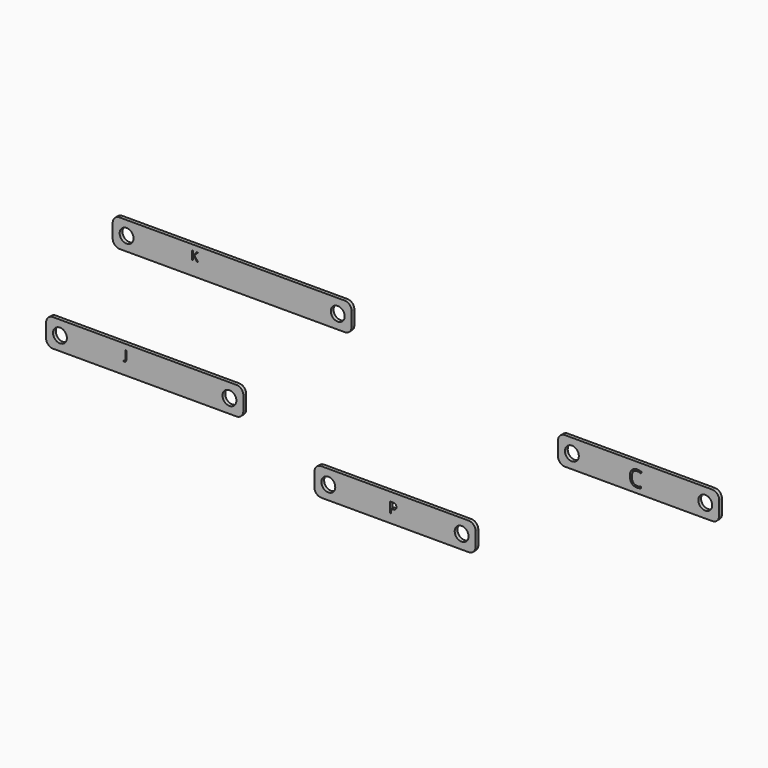
from build123d import *

# Parameters (mm, degrees)
F1_R     = 6.35
F2_DEPTH = 3.175
F3_R     = 6.35
F4_DEPTH = 3.175
F5_R     = 6.35
F6_DEPTH = 3.175
F7_R     = 6.35
F8_DEPTH = 3.175


# Not quite as in the source:
# - a length typed as a fraction of an inch, garbled in the dataset ("3 / 203.2 mm" for 3/8 in), is restored


with BuildPart() as f2:
    # F1 (on Front) → F2 (new body)
    with BuildSketch(Plane.XZ):
        with BuildLine():
            Line((95.5763677621, 23.3495529922), (-110.1636322379, 23.3495529922))
            ThreePointArc((-110.1636322379, 23.3495529922), (-114.6537602984, 21.4896810527), (-116.5136322379, 16.9995529922))
            Line((-116.5136322379, 16.9995529922), (-116.5136322379, 4.2995529922))
            ThreePointArc((-116.5136322379, 4.2995529922), (-114.6537602984, -0.1905750684), (-110.1636322379, -2.0504470078))
            Line((-110.1636322379, -2.0504470078), (95.5763677621, -2.0504470078))
            ThreePointArc((95.5763677621, -2.0504470078), (100.0664958226, -0.1905750684), (101.9263677621, 4.2995529922))
            Line((101.9263677621, 4.2995529922), (101.9263677621, 16.9995529922))
            ThreePointArc((101.9263677621, 16.9995529922), (100.0664958226, 21.4896810527), (95.5763677621, 23.3495529922))
        make_face()
        with Locations((-103.8136322379, 10.6495529922)):
            Circle(F1_R, mode=Mode.SUBTRACT)
        Polygon((-41.6826481417, 14.9866065492), (-38.4835676154, 10.6495529922), (-39.5325840524, 10.6495529922), (-42.3271638406, 14.3689456712), (-43.1311300379, 13.655614494), (-43.1311300379, 10.6495529922), (-44.0223744027, 10.6495529922), (-44.0223744027, 18.3182827531), (-43.1311300379, 18.3182827531), (-43.1311300379, 14.5149687592), (-39.653430746, 18.3182827531), (-38.5993790301, 18.3182827531), align=None, mode=Mode.SUBTRACT)
        with Locations((89.2263677621, 10.6495529922)):
            Circle(F1_R, mode=Mode.SUBTRACT)
    extrude(amount=F2_DEPTH)


with BuildPart() as f4:
    # F3 (on Front) → F4 (new body)
    with BuildSketch(Plane.XZ):
        with BuildLine():
            Line((-3.4336355138, -76.6887728453), (-171.0736355138, -76.6887728453))
            ThreePointArc((-171.0736355138, -76.6887728453), (-175.5637635743, -78.5486447847), (-177.4236355138, -83.0387728453))
            Line((-177.4236355138, -83.0387728453), (-177.4236355138, -95.7387728453))
            ThreePointArc((-177.4236355138, -95.7387728453), (-175.5637635743, -100.2289009058), (-171.0736355138, -102.0887728453))
            Line((-171.0736355138, -102.0887728453), (-3.4336355138, -102.0887728453))
            ThreePointArc((-3.4336355138, -102.0887728453), (1.0564925468, -100.2289009058), (2.9163644862, -95.7387728453))
            Line((2.9163644862, -95.7387728453), (2.9163644862, -83.0387728453))
            ThreePointArc((2.9163644862, -83.0387728453), (1.0564925468, -78.5486447847), (-3.4336355138, -76.6887728453))
        make_face()
        with Locations((-9.7836355138, -89.3887728453)):
            Circle(F3_R, mode=Mode.SUBTRACT)
        with Locations((-164.7236355138, -89.3887728453)):
            Circle(F3_R, mode=Mode.SUBTRACT)
        with BuildLine():
            add(Edge.make_bspline(
                [(-104.6017276977, -90.8599134965), (-105.1052555874, -91.4079196832), (-106.0502095939, -91.4079196832)],
                knots=[0, 0, 0, 1, 1, 1], degree=2))
            add(Edge.make_bspline(
                [(-106.0502095939, -91.4079196832), (-106.5419884995, -91.4079196832), (-106.8256425441, -91.266931874)],
                knots=[0, 0, 0, 1, 1, 1], degree=2))
            Line((-106.8256425441, -91.266931874), (-106.8256425441, -90.5066047605))
            add(Edge.make_bspline(
                [(-106.8256425441, -90.5066047605), (-106.4530319057, -90.6106671911), (-106.0502095939, -90.6106671911)],
                knots=[0, 0, 0, 1, 1, 1], degree=2))
            add(Edge.make_bspline(
                [(-106.0502095939, -90.6106671911), (-105.5298974411, -90.6106671911), (-105.2596708069, -90.29596226)],
                knots=[0, 0, 0, 1, 1, 1], degree=2))
            add(Edge.make_bspline(
                [(-105.2596708069, -90.29596226), (-104.9894441728, -89.9812573289), (-104.9894441728, -89.3887728453)],
                knots=[0, 0, 0, 1, 1, 1], degree=2))
            Line((-104.9894441728, -89.3887728453), (-104.9894441728, -81.7200430843))
            Line((-104.9894441728, -81.7200430843), (-104.0981998079, -81.7200430843))
            Line((-104.0981998079, -81.7200430843), (-104.0981998079, -89.3149220881))
            add(Edge.make_bspline(
                [(-104.0981998079, -89.3149220881), (-104.0981998079, -90.3119073098), (-104.6017276977, -90.8599134965)],
                knots=[0, 0, 0, 1, 1, 1], degree=2))
        make_face(mode=Mode.SUBTRACT)
    extrude(amount=F4_DEPTH)


with BuildPart() as f6:
    # F5 (on Front) → F6 (new body)
    with BuildSketch(Plane.XZ):
        with BuildLine():
            Line((208.8844542503, -116.8920610428), (74.2644542503, -116.8920610428))
            ThreePointArc((74.2644542503, -116.8920610428), (69.7743261898, -118.7519329823), (67.9144542503, -123.2420610428))
            Line((67.9144542503, -123.2420610428), (67.9144542503, -135.9420610428))
            ThreePointArc((67.9144542503, -135.9420610428), (69.7743261898, -140.4321891033), (74.2644542503, -142.2920610428))
            Line((74.2644542503, -142.2920610428), (208.8844542503, -142.2920610428))
            ThreePointArc((208.8844542503, -142.2920610428), (213.3745823109, -140.4321891033), (215.2344542503, -135.9420610428))
            Line((215.2344542503, -135.9420610428), (215.2344542503, -123.2420610428))
            ThreePointArc((215.2344542503, -123.2420610428), (213.3745823109, -118.7519329823), (208.8844542503, -116.8920610428))
        make_face()
        with Locations((202.5344542503, -129.5920610428)):
            Circle(F5_R, mode=Mode.SUBTRACT)
        with Locations((80.6144542503, -129.5920610428)):
            Circle(F5_R, mode=Mode.SUBTRACT)
        with BuildLine():
            add(Edge.make_bspline(
                [(139.3608329236, -124.7941682377), (142.9005294922, -124.7941682377), (142.9005294922, -127.5461169134)],
                knots=[0, 0, 0, 1, 1, 1], degree=2))
            add(Edge.make_bspline(
                [(142.9005294922, -127.5461169134), (142.9005294922, -128.9810172748), (141.9215304704, -129.7532583194)],
                knots=[0, 0, 0, 1, 1, 1], degree=2))
            add(Edge.make_bspline(
                [(141.9215304704, -129.7532583194), (140.9425314487, -130.525499364), (139.1209936701, -130.525499364)],
                knots=[0, 0, 0, 1, 1, 1], degree=2))
            Line((139.1209936701, -130.525499364), (138.0086357531, -130.525499364))
            Line((138.0086357531, -130.525499364), (138.0086357531, -134.2409402132))
            Line((138.0086357531, -134.2409402132), (136.9107508945, -134.2409402132))
            Line((136.9107508945, -134.2409402132), (136.9107508945, -124.7941682377))
            Line((136.9107508945, -124.7941682377), (139.3608329236, -124.7941682377))
        make_face(mode=Mode.SUBTRACT)
    extrude(amount=F6_DEPTH)


with BuildPart() as f8:
    # F7 (on Front) → F8 (new body)
    with BuildSketch(Plane.XZ):
        with BuildLine():
            Line((431.5898662186, -19.4524478495), (296.9698662186, -19.4524478495))
            ThreePointArc((296.9698662186, -19.4524478495), (292.479738158, -21.312319789), (290.6198662186, -25.8024478495))
            Line((290.6198662186, -25.8024478495), (290.6198662186, -38.5024478495))
            ThreePointArc((290.6198662186, -38.5024478495), (292.479738158, -42.99257591), (296.9698662186, -44.8524478495))
            Line((296.9698662186, -44.8524478495), (431.5898662186, -44.8524478495))
            ThreePointArc((431.5898662186, -44.8524478495), (436.0799942791, -42.99257591), (437.9398662186, -38.5024478495))
            Line((437.9398662186, -38.5024478495), (437.9398662186, -25.8024478495))
            ThreePointArc((437.9398662186, -25.8024478495), (436.0799942791, -21.312319789), (431.5898662186, -19.4524478495))
        make_face()
        with BuildLine():
            add(Edge.make_bspline(
                [(366.4639369183, -27.8038420737), (364.8282573372, -27.0380036572), (363.1925777562, -27.0380036572)],
                knots=[0, 0, 0, 1, 1, 1], degree=2))
            add(Edge.make_bspline(
                [(363.1925777562, -27.0380036572), (360.8194241444, -27.0380036572), (359.4453272324, -28.6185302658)],
                knots=[0, 0, 0, 1, 1, 1], degree=2))
            add(Edge.make_bspline(
                [(359.4453272324, -28.6185302658), (358.0712303204, -30.1990568745), (358.0712303204, -32.9472506985)],
                knots=[0, 0, 0, 1, 1, 1], degree=2))
            add(Edge.make_bspline(
                [(358.0712303204, -32.9472506985), (358.0712303204, -35.7710828846), (359.3964774569, -37.3137903122)],
                knots=[0, 0, 0, 1, 1, 1], degree=2))
            add(Edge.make_bspline(
                [(359.3964774569, -37.3137903122), (360.7217245933, -38.8564977398), (363.1736681657, -38.8564977398)],
                knots=[0, 0, 0, 1, 1, 1], degree=2))
            add(Edge.make_bspline(
                [(363.1736681657, -38.8564977398), (364.6801322114, -38.8564977398), (366.6120620441, -38.3144228112)],
                knots=[0, 0, 0, 1, 1, 1], degree=2))
            Line((366.6120620441, -38.3144228112), (366.6120620441, -39.7799160775))
            add(Edge.make_bspline(
                [(366.6120620441, -39.7799160775), (365.1150527937, -40.344052195), (362.9183886935, -40.344052195)],
                knots=[0, 0, 0, 1, 1, 1], degree=2))
            add(Edge.make_bspline(
                [(362.9183886935, -40.344052195), (359.7384258857, -40.344052195), (358.0097741512, -38.4121223623)],
                knots=[0, 0, 0, 1, 1, 1], degree=2))
            add(Edge.make_bspline(
                [(358.0097741512, -38.4121223623), (356.2811224167, -36.4801925296), (356.2811224167, -32.9251895095)],
                knots=[0, 0, 0, 1, 1, 1], degree=2))
            add(Edge.make_bspline(
                [(356.2811224167, -32.9251895095), (356.2811224167, -30.7001610236), (357.1131444001, -29.0266622615)],
                knots=[0, 0, 0, 1, 1, 1], degree=2))
            add(Edge.make_bspline(
                [(357.1131444001, -29.0266622615), (357.9451663835, -27.3531634994), (359.5162381969, -26.447078953)],
                knots=[0, 0, 0, 1, 1, 1], degree=2))
            add(Edge.make_bspline(
                [(359.5162381969, -26.447078953), (361.0873100103, -25.5409944067), (363.2146389452, -25.5409944067)],
                knots=[0, 0, 0, 1, 1, 1], degree=2))
            add(Edge.make_bspline(
                [(363.2146389452, -25.5409944067), (365.4774866122, -25.5409944067), (367.1730465632, -26.3667131933)],
                knots=[0, 0, 0, 1, 1, 1], degree=2))
            Line((367.1730465632, -26.3667131933), (366.4639369183, -27.8038420737))
        make_face(mode=Mode.SUBTRACT)
        with Locations((425.2398662186, -32.1524478495)):
            Circle(F7_R, mode=Mode.SUBTRACT)
        with Locations((303.3198662186, -32.1524478495)):
            Circle(F7_R, mode=Mode.SUBTRACT)
    extrude(amount=F8_DEPTH)


solid = Compound([f2.part, f4.part, f6.part, f8.part])
